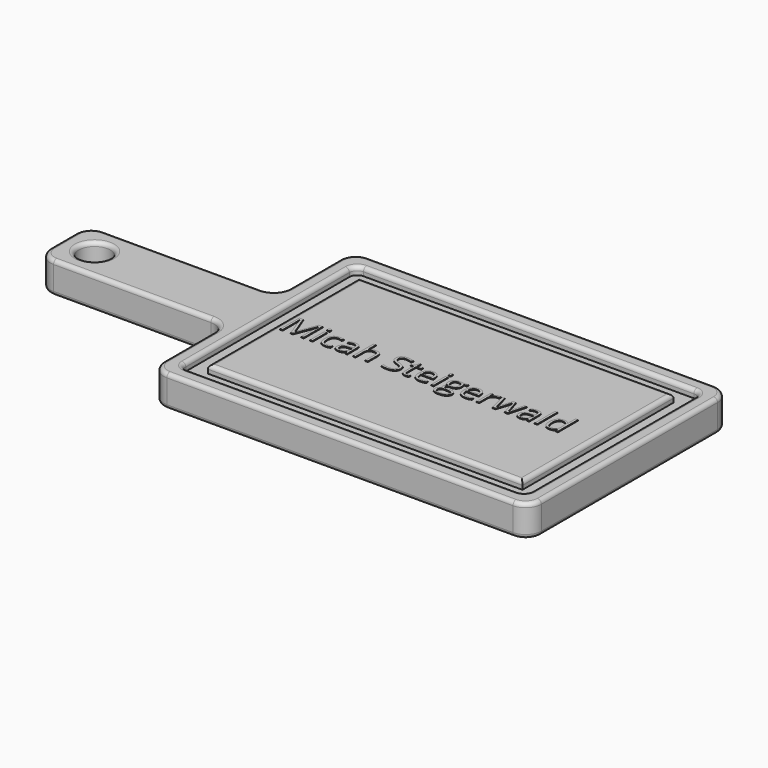
from build123d import *

# Parameters (mm, degrees)
F0_W         = 152.4
F0_H         = 50.8
F1_DEPTH     = 25.4
F2_R         = 12.7
F3_DEPTH     = 25.4
F5_DEPTH     = 6.35
F6_R         = 6.35
F7_R         = 12.7
F8_R         = 3.175
F9_TEXT_SIZE = 26.9789227166
F10_DEPTH    = 0.508


# Not quite as in the source:
# - Text() gives the source's letters only with a copy of the font that has no kerning and outlines rounded to 1/6400 em; it was checked with that copy


with BuildPart() as f1:
    # F0 (on Top) → F1 (new body)
    with BuildSketch(Plane.XY):
        Polygon((0, 76.2), (0, 0), (304.8, 0), (304.8, 203.2), (0, 203.2), (0, 127), align=None)
        with Locations((-76.2, 101.6)):
            Rectangle(F0_W, F0_H)
    extrude(amount=F1_DEPTH)

    # F2 (on face) → F3 (cut)
    with BuildSketch(Plane.XY.offset(25.4)):
        with Locations((-127, 101.6)):
            Circle(F2_R)
    extrude(amount=-F3_DEPTH, mode=Mode.SUBTRACT)

    # F4 (on face) → F5 (cut)
    with BuildSketch(Plane.XY.offset(25.4)):
        Polygon((12.6999939203, 76.2), (12.6999939203, 12.6999939203), (292.1000060797, 12.6999939203), (292.1000060797, 190.5000060797), (12.6999939203, 190.5000060797), (12.6999939203, 127), align=None)
        Polygon((25.4000002861, 76.2), (25.4000002861, 127), (25.4000002861, 177.7999997139), (279.3999997139, 177.7999997139), (279.3999997139, 25.4000002861), (25.4000002861, 25.4000002861), align=None, mode=Mode.SUBTRACT)
    extrude(amount=-F5_DEPTH, mode=Mode.SUBTRACT)

    # F6
    f6_edges = [f1.edges().sort_by_distance(p)[0] for p in [
        (12.699994, 190.500006, 22.225),
        (12.699994, 12.699994, 22.225),
        (292.100006, 12.699994, 22.225),
        (292.100006, 190.500006, 22.225),
    ]]
    fillet(f6_edges, radius=F6_R)

    # F7
    f7_edges = [f1.edges().sort_by_distance(p)[0] for p in [
        (-152.4, 76.2, 12.7),
        (0, 0, 12.7),
        (-152.4, 127, 12.7),
        (0, 127, 12.7),
        (0, 203.2, 12.7),
        (0, 76.2, 12.7),
        (304.8, 0, 12.7),
        (304.8, 203.2, 12.7),
    ]]
    fillet(f7_edges, radius=F7_R)

    # F8
    f8_edges = [f1.edges().sort_by_distance(p)[0] for p in [
        (152.4, 177.8, 25.4),
        (279.4, 101.6, 25.4),
        (152.4, 25.4, 25.4),
        (25.4, 101.6, 25.4),
        (0, 38.1, 25.4),
        (-3.719744, 72.480256, 25.4),
        (3.719744, 3.719744, 25.4),
        (-76.2, 76.2, 25.4),
        (152.4, 0, 25.4),
        (-148.680256, 79.919744, 25.4),
        (301.080256, 3.719744, 25.4),
        (-152.4, 101.6, 25.4),
        (304.8, 101.6, 25.4),
        (-148.680256, 123.280256, 25.4),
        (301.080256, 199.480256, 25.4),
        (-76.2, 127, 25.4),
        (152.4, 203.2, 25.4),
        (-3.719744, 130.719744, 25.4),
        (3.719744, 199.480256, 25.4),
        (0, 165.1, 25.4),
        (152.4, 12.699994, 25.4),
        (14.559866, 14.559866, 25.4),
        (290.240134, 14.559866, 25.4),
        (12.699994, 101.6, 25.4),
        (292.100006, 101.6, 25.4),
        (14.559866, 188.640134, 25.4),
        (290.240134, 188.640134, 25.4),
        (152.4, 190.500006, 25.4),
        (-139.7, 101.6, 25.4),
        (0, 38.1, 0),
        (-3.719744, 72.480256, 0),
        (3.719744, 3.719744, 0),
        (-76.2, 76.2, 0),
        (152.4, 0, 0),
        (-148.680256, 79.919744, 0),
        (301.080256, 3.719744, 0),
        (-152.4, 101.6, 0),
        (304.8, 101.6, 0),
        (-148.680256, 123.280256, 0),
        (301.080256, 199.480256, 0),
        (-76.2, 127, 0),
        (152.4, 203.2, 0),
        (-3.719744, 130.719744, 0),
        (3.719744, 199.480256, 0),
        (0, 165.1, 0),
        (-139.7, 101.6, 0),
    ]]
    fillet(f8_edges, radius=F8_R)

    # F9 (on face) → F10 (join)
    with BuildSketch(Plane.XY.offset(25.4)):
        with Locations((28.5750002861, 91.1460146308)):
            Text('Micah Steigerwald', F9_TEXT_SIZE, font='Open Sans', text_align=(TextAlign.LEFT, TextAlign.BOTTOM))
    extrude(amount=F10_DEPTH)


solid = f1.part
